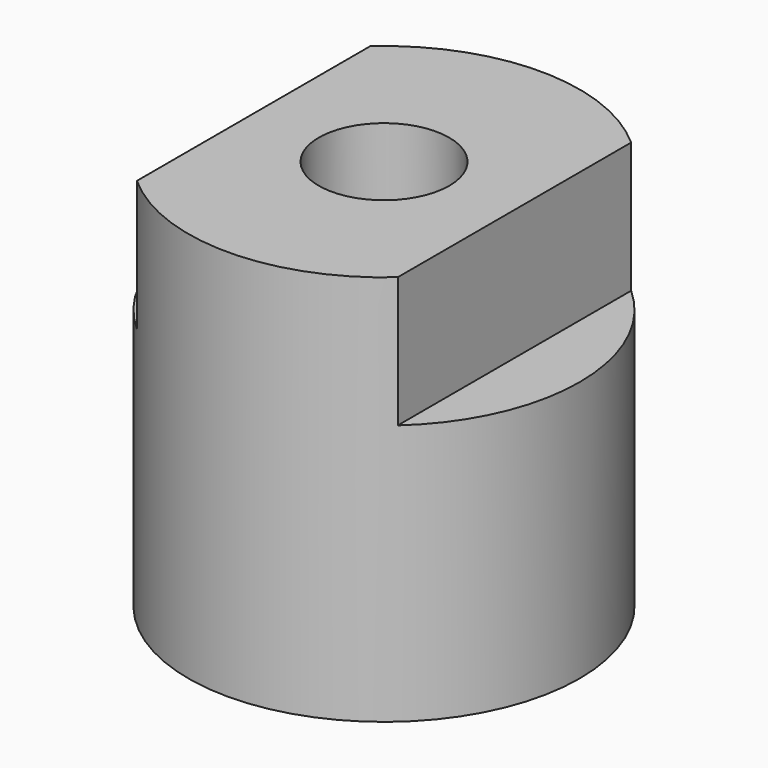
from build123d import *

# Parameters (mm, degrees)
F0_R     = 30
F1_DEPTH = 60
F2_W     = 10
F2_H     = 20
F3_DEPTH = 50
F4_R     = 15
F5_DEPTH = 25
F6_R     = 10
F7_DEPTH = 100
F8_SIZE  = 4.99999


# Not quite as in the source:
# - a fillet or chamfer is up to 0.001 mm smaller than in the source, because OpenCascade refuses the exact size


with BuildPart() as f1:
    # F0 (on Top) → F1 (new body)
    with BuildSketch(Plane.XY):
        Circle(F0_R)
    extrude(amount=F1_DEPTH)

    # F2 (on Front) → F3 (cut, symmetric)
    with BuildSketch(Plane.XZ):
        with Locations((-25, 50)):
            Rectangle(F2_W, F2_H)
        with Locations((25, 50)):
            Rectangle(F2_W, F2_H)
    extrude(amount=F3_DEPTH, both=True, mode=Mode.SUBTRACT)

    # F4 (on face) → F5 (cut)
    with BuildSketch(Plane(origin=(0, 0, 0), x_dir=(1, 0, 0), z_dir=(0, 0, -1))):
        Circle(F4_R)
    extrude(amount=-F5_DEPTH, mode=Mode.SUBTRACT)

    # F6 (on face) → F7 (cut)
    with BuildSketch(Plane.XY.offset(60)):
        Circle(F6_R)
    extrude(amount=-F7_DEPTH, mode=Mode.SUBTRACT)

    # F8 (size 5 in the source; OpenCascade refuses exactly that, so slightly less here)
    f8_edges = [f1.edges().sort_by_distance(p)[0] for p in [
        (-10, 0, 25),
    ]]
    chamfer(f8_edges, length=F8_SIZE)


solid = f1.part
